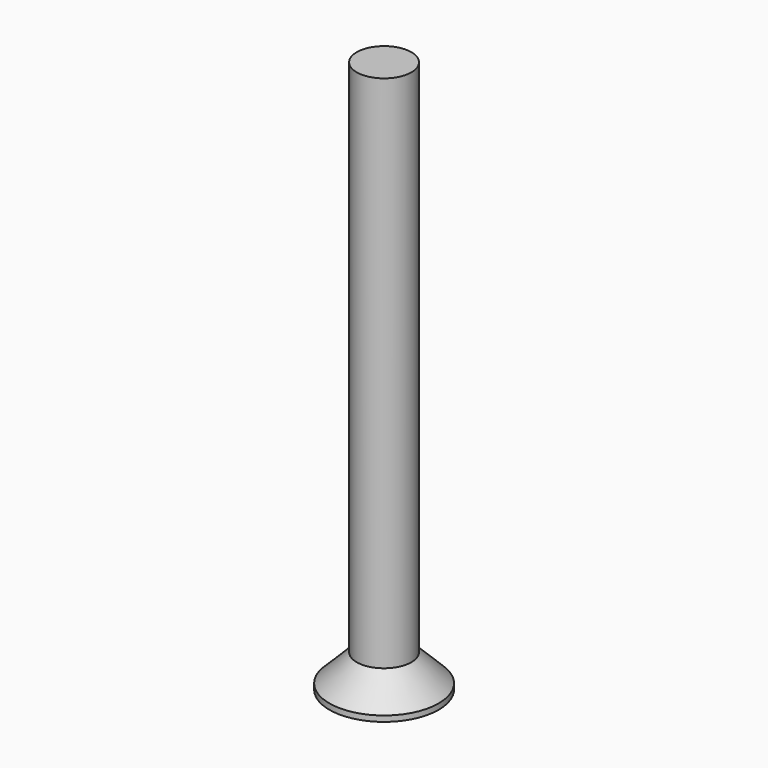
from build123d import *

# Parameters (mm, degrees)
F0_R        = 1.45
F1_DEPTH    = 27.5
F2_R        = 2.9
F3_DEPTH    = 1.8
F4_W        = 1
F4_H        = 1
F5_DEPTH    = 1.5
F6_S5_R     = 1.45
F6_T6_DEPTH = 6


# Not quite as in the source:
# - a fillet or chamfer that OpenCascade refuses, or shapes differently, is made with other operations: its cross-section is extruded or revolved along the edge and cut away or added


with BuildPart() as f1:
    # F0 (on Top) → F1 (new body)
    with BuildSketch(Plane.XY):
        Circle(F0_R)
    extrude(amount=F1_DEPTH)

    # F2 (on Top) → F3 (join)
    with BuildSketch(Plane.XY):
        Circle(F2_R)
    extrude(amount=-F3_DEPTH)

    # F4 (on face) → F5 (cut)
    with BuildSketch(Plane(origin=(0, 0, -1.8), x_dir=(1, 0, 0), z_dir=(0, 0, -1))):
        with Locations((1, 0)):
            Rectangle(F4_W, F4_H)
        Rectangle(F4_W, F4_H)
        with Locations((0, 1)):
            Rectangle(F4_W, F4_H)
        with Locations((-1, 0)):
            Rectangle(F4_W, F4_H)
        with Locations((0, -1)):
            Rectangle(F4_W, F4_H)
    extrude(amount=-F5_DEPTH, mode=Mode.SUBTRACT)

    # F6: chamfer of 1.5 on 1 edges, made by hand


with BuildPart() as f6_tool2:
    # F6_s3 → F6_t4 (revolve)
    with BuildSketch(Plane.XZ):
        Polygon((2.9, -1.5), (1.4, 0), (2.9, 0), align=None)
    revolve(axis=Axis((0, 0, 0), (0, 0, 1)))

    # F6_s5 → F6_t6 (cut, symmetric)
    with BuildSketch(Plane.XY.offset(-0.7)):
        Circle(F6_S5_R)
    extrude(amount=F6_T6_DEPTH, both=True, mode=Mode.SUBTRACT)


with BuildPart() as f1_1:
    add(f1.part)

    # F6_t1: cut F6_tool2
    add(f6_tool2.part, mode=Mode.SUBTRACT)


solid = f1_1.part
